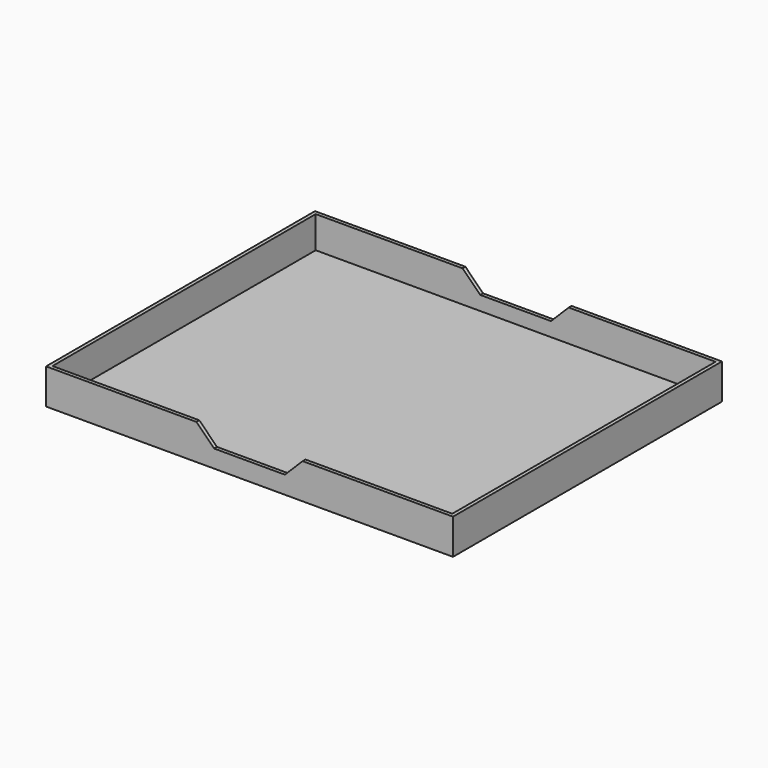
from build123d import *

# Parameters (mm, degrees)
F1_DEPTH = 190
F2_W     = 230
F2_H     = 20
F3_DEPTH = 2
F6_DEPTH = 190.001


# Not quite as in the source:
# - a pattern or mirror of a feature is missing from the dataset's text; its kind, count and spacing are read off the source's solid


with BuildPart() as f1:
    # F0 (on Front) → F1 (new body)
    with BuildSketch(Plane.XZ):
        Polygon((-115, 10), (-115, -10), (115, -10), (115, 10), (113, 10), (113, -8), (-113, -8), (-113, 10), align=None)
    extrude(amount=F1_DEPTH)

    # F2 (on face) → F3 (join)
    with BuildSketch(Plane.XZ.offset(190)):
        Rectangle(F2_W, F2_H)
    f3 = extrude(amount=-F3_DEPTH)

    # F3_copies: F3 across plane
    add(f3.mirror(Plane.ZX.offset(-95)))

    # F5 (on face) → F6 (cut, through all)
    with BuildSketch(Plane.XZ.offset(190)):
        Polygon((-20, 0), (0, 0), (20, 0), (30, 10), (0, 10), (-30, 10), align=None)
    extrude(amount=-F6_DEPTH, mode=Mode.SUBTRACT)


solid = f1.part
